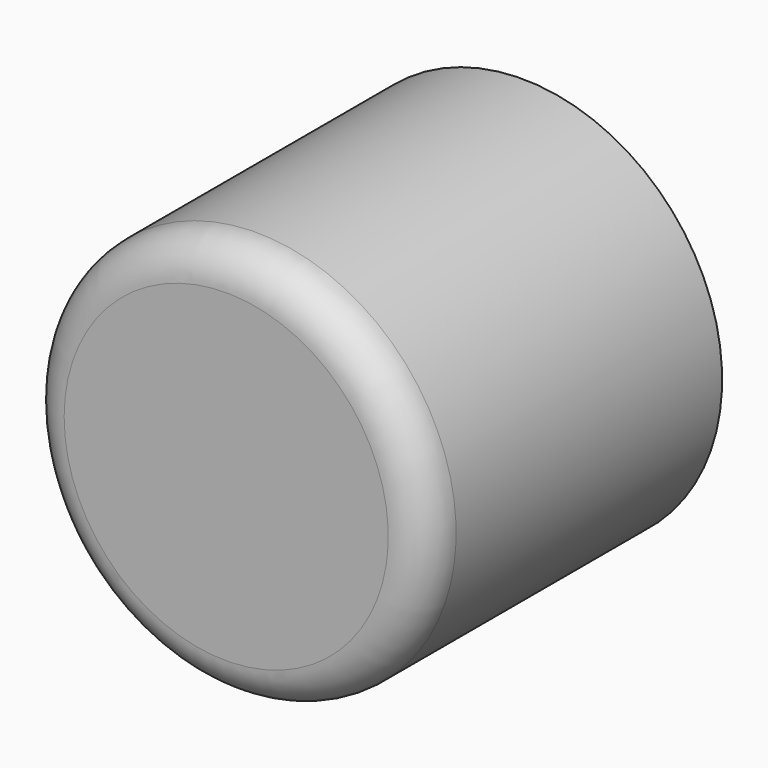
from build123d import *

# Parameters (mm, degrees)
F0_W     = 23.4204549342
F0_H     = 2.8636362404
F3_R     = 5
F5_W     = 35.1818175986
F5_H     = 36.409093067
F6_DEPTH = 64


# Not quite as in the source:
# - a fillet or chamfer that OpenCascade refuses, or shapes differently, is made with other operations: its cross-section is extruded or revolved along the edge and cut away or added


with BuildPart() as f1:
    # F0 (on Top) → F1 (revolve)
    with BuildSketch(Plane.XY):
        Polygon((-23.4204549342, 28.6363661289), (-26.4886375517, 28.6363661289), (-26.4886375517, -20.4545464367), (-23.4204549342, -20.4545464367), (-23.4204549342, -17.5909101963), align=None)
        with Locations((-11.7102274671, -19.0227283165)):
            Rectangle(F0_W, F0_H)
    revolve(axis=Axis((0, -19.0227283165, 0), (0, 1, 0)))

    # F3
    f3_edges = [f1.edges().sort_by_distance(p)[0] for p in [
        (26.488638, -20.454546, 0),
    ]]
    fillet(f3_edges, radius=F3_R)

    # F4: fillet of radius 5 on 1 edges, made by hand

    # F4_s1 → F4_t2 (revolve, cut)
    with BuildSketch(Plane.XY):
        with BuildLine():
            ThreePointArc((-26.4886375517, 28.6363661289), (-24.2575781097, 26.7941920001), (-23.4204549342, 24.0246330924))
            Line((-23.4204549342, 24.0246330924), (-23.4204549342, 28.6363661289))
            Line((-23.4204549342, 28.6363661289), (-26.4886375517, 28.6363661289))
        make_face()
    revolve(axis=Axis((0, 28.6363661289, 0), (0, 1, 0)), mode=Mode.SUBTRACT)

    # F5 (on offset) → F6 (cut)
    with BuildSketch(Plane.YZ.offset(-26.45)):
        with Locations((7.4659097008, -1.0227272287)):
            Rectangle(F5_W, F5_H)
    extrude(amount=-F6_DEPTH, mode=Mode.SUBTRACT)


solid = f1.part
